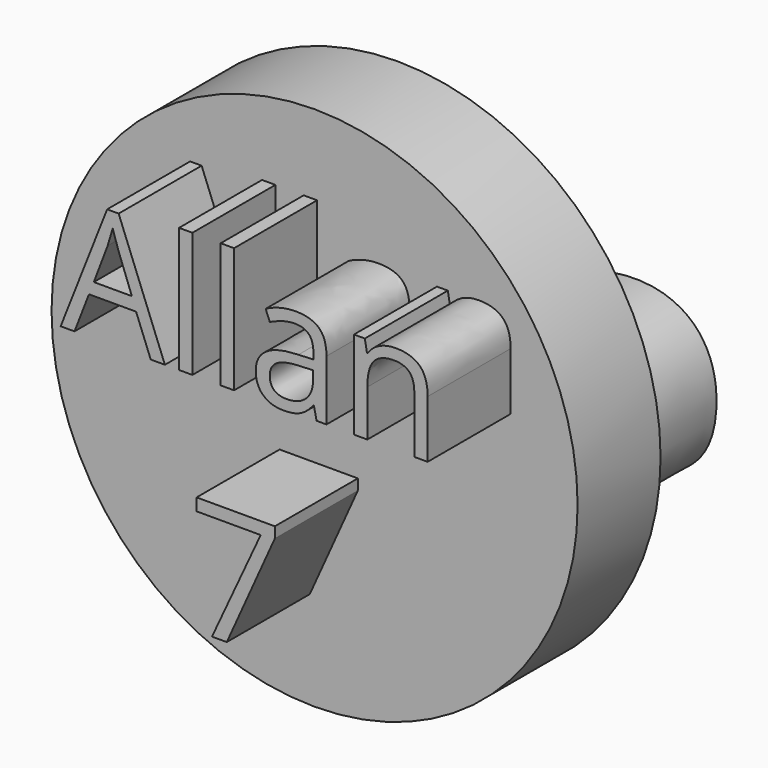
from build123d import *

# Parameters (mm, degrees)
F0_R         = 64.4114707055
F1_DEPTH     = 25.4
F2_TEXT_SIZE = 40.3332278236
F3_DEPTH     = 25.4
F4_TEXT_SIZE = 53.9630806694
F5_DEPTH     = 25.4


# Not quite as in the source:
# - Text() gives the source's letters only with a copy of the font that has no kerning and outlines rounded to 1/6400 em; it was checked with that copy


with BuildPart() as f1:
    # F0 (on Front) → F1 (new body)
    with BuildSketch(Plane.XZ):
        Circle(F0_R)
    extrude(amount=F1_DEPTH)

    # F2 (on face) → F3 (join)
    with BuildSketch(Plane.XZ.offset(25.4)):
        with Locations((-41.857548058, 14.3196871504)):
            Text('Allan', F2_TEXT_SIZE, font='Open Sans', text_align=(TextAlign.LEFT, TextAlign.BOTTOM))
        with Locations((-10.4165365562, -40.5335026897)):
            Text('7', F2_TEXT_SIZE, font='Open Sans', text_align=(TextAlign.LEFT, TextAlign.BOTTOM))
    extrude(amount=F3_DEPTH)

    # F4 (on face) → F5 (join)
    with BuildSketch(Plane(origin=(0, 0, 0), x_dir=(-1, 0, 0), z_dir=(0, 1, 0))):
        with Locations((-61.0839799047, -19.5268476382)):
            Text('Goat', F4_TEXT_SIZE, font='Open Sans', text_align=(TextAlign.LEFT, TextAlign.BOTTOM))
    extrude(amount=F5_DEPTH)


solid = f1.part
